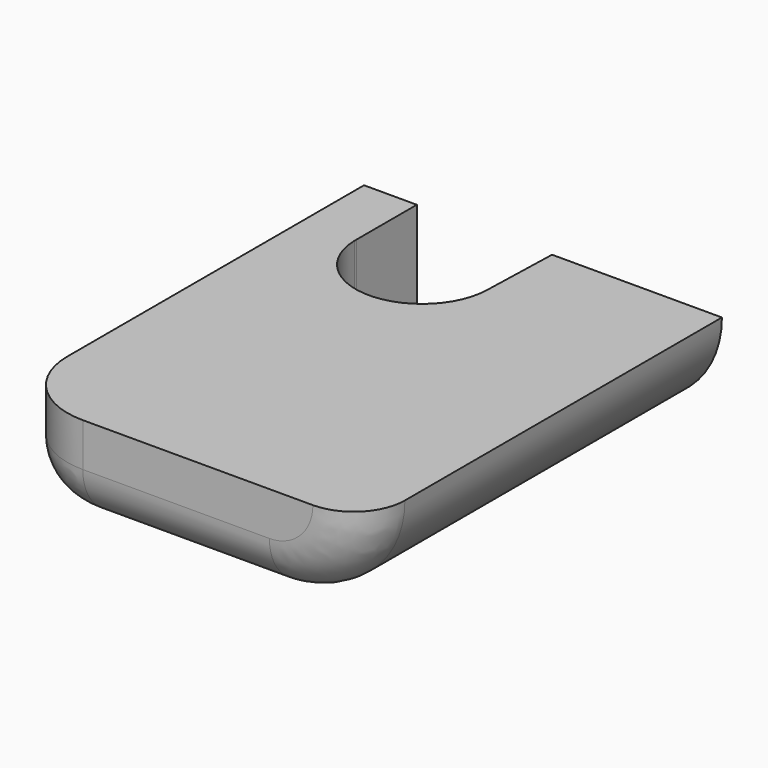
from build123d import *

# Parameters (mm, degrees)
F0_W         = 14
F0_H         = 17.5
F1_DEPTH     = 3.7
F3_DEPTH     = 5.4
F4_R         = 3.69999
F5_R         = 3
F6_T1_DEPTH  = 7.30001
F6_T3_DEPTH  = 5.00001
F6_T5_DEPTH  = 19.5
F6_T8_ANGLE  = 90
F6_T10_ANGLE = 90


# Not quite as in the source:
# - a fillet or chamfer that OpenCascade refuses, or shapes differently, is made with other operations: its cross-section is extruded or revolved along the edge and cut away or added
# - a fillet or chamfer is up to 0.001 mm smaller than in the source, because OpenCascade refuses the exact size


with BuildPart() as f1:
    # F0 (on Top) → F1 (new body)
    with BuildSketch(Plane.XY):
        with Locations((-0.4103374667, 3.4223956802)):
            Rectangle(F0_W, F0_H)
    extrude(amount=F1_DEPTH)

    # F2 (on face) → F3 (cut)
    with BuildSketch(Plane.XY.offset(3.7)):
        with BuildLine():
            Line((-5.3451164257, 9.1307080224), (-5.3451164257, 9.2324278445))
            ThreePointArc((-5.3451164257, 9.2324278445), (-5.3456139214, 9.1815679334), (-5.3451164257, 9.1307080224))
        make_face()
        with BuildLine():
            Line((-5.3451164257, 12.1723956802), (-5.3451164257, 9.2324278445))
            Line((-5.3451164257, 9.2324278445), (-5.3451164257, 9.1307080224))
            ThreePointArc((-5.3451164257, 9.1307080224), (-2.7588797704, 6.5816017765), (-0.1467657558, 9.1041843944))
            Line((-0.1467657558, 9.1041843944), (-0.055406418, 12.1723956802))
            Line((-0.055406418, 12.1723956802), (-5.3451164257, 12.1723956802))
        make_face()
    extrude(amount=-F3_DEPTH, mode=Mode.SUBTRACT)

    # F4 (radius 3.7 in the source; OpenCascade refuses exactly that, so slightly less here)
    f4_edges = [f1.edges().sort_by_distance(p)[0] for p in [
        (6.589663, 3.422396, 0),
    ]]
    fillet(f4_edges, radius=F4_R)

    # F5
    f5_edges = [f1.edges().sort_by_distance(p)[0] for p in [
        (-7.410337, -5.327604, 1.85),
    ]]
    fillet(f5_edges, radius=F5_R)

    # F6: fillet of radius 2 on 1 edges, made by hand

    # F6_s2 → F6_t1 (cut)
    with BuildSketch(Plane.YZ.offset(-4.4103374667)):
        with BuildLine():
            ThreePointArc((-5.3276043198, 2), (-4.7418178821, 0.5857864376), (-3.3276043198, 0))
            Line((-3.3276043198, 0), (-5.3276043198, 0))
            Line((-5.3276043198, 0), (-5.3276043198, 2))
        make_face()
    extrude(amount=F6_T1_DEPTH, mode=Mode.SUBTRACT)

    # F6_s4 → F6_t3 (cut)
    with BuildSketch(Plane.XY.offset(3.69999)):
        with BuildLine():
            ThreePointArc((4.5896625333, -5.3276043198), (6.0038760956, -4.7418178821), (6.5896625333, -3.3276043198))
            Line((6.5896625333, -3.3276043198), (6.5896625333, -5.3276043198))
            Line((6.5896625333, -5.3276043198), (4.5896625333, -5.3276043198))
        make_face()
    extrude(amount=F6_T3_DEPTH, mode=Mode.SUBTRACT)

    # F6_s6 → F6_t5 (cut)
    with BuildSketch(Plane.XZ.offset(-17.1723956802)):
        with BuildLine():
            ThreePointArc((-5.4103374667, 0), (-6.8245510291, 0.5857864376), (-7.4103374667, 2))
            Line((-7.4103374667, 2), (-7.4103374667, 0))
            Line((-7.4103374667, 0), (-5.4103374667, 0))
        make_face()
    extrude(amount=F6_T5_DEPTH, mode=Mode.SUBTRACT)

    # F6_s7 → F6_t8 (revolve, cut)
    with BuildSketch(Plane.YZ.offset(2.8896725333)):
        with BuildLine():
            ThreePointArc((-5.3276043198, 2), (-4.7418178821, 0.5857864376), (-3.3276043198, 0))
            Line((-3.3276043198, 0), (-5.3276043198, 0))
            Line((-5.3276043198, 0), (-5.3276043198, 2))
        make_face()
    revolve(axis=Axis((2.8896725333, -5.3276043198, 3.69999), (0, -1, 0)), revolution_arc=F6_T8_ANGLE, mode=Mode.SUBTRACT)

    # F6_s9 → F6_t10 (revolve, cut)
    with BuildSketch(Plane.YZ.offset(-4.4103374667)):
        with BuildLine():
            ThreePointArc((-5.3276043198, 2), (-4.7418178821, 0.5857864376), (-3.3276043198, 0))
            Line((-3.3276043198, 0), (-5.3276043198, 0))
            Line((-5.3276043198, 0), (-5.3276043198, 2))
        make_face()
    revolve(axis=Axis((-4.4103374667, -2.3276043198, 0), (0, 0, -1)), revolution_arc=F6_T10_ANGLE, mode=Mode.SUBTRACT)


solid = f1.part
